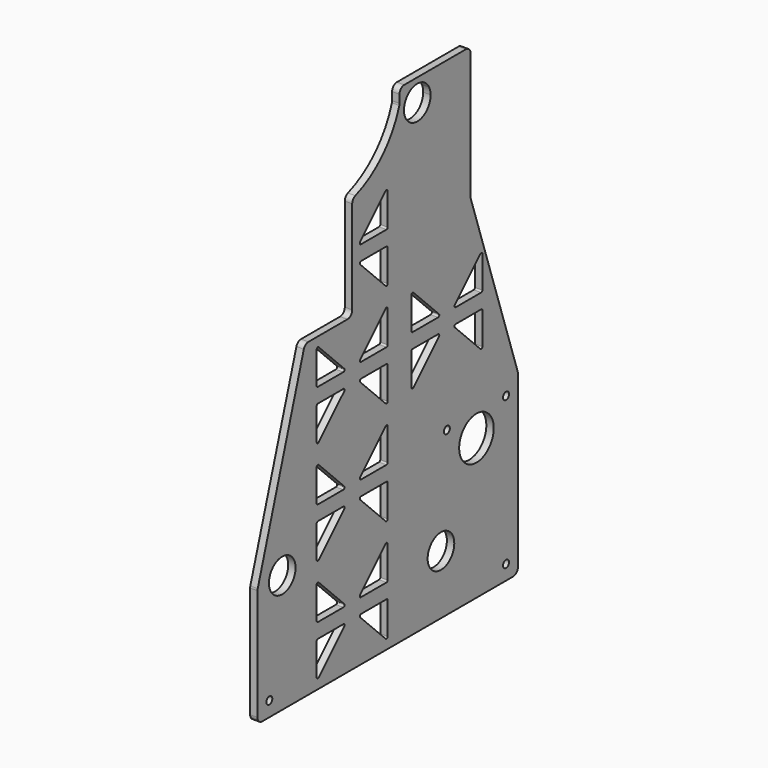
from build123d import *

# Parameters (mm, degrees)
F0_R     = 3.175
F0_R_2   = 14.2875
F0_R_3   = 18.542
F1_DEPTH = 6.35
F2_R     = 5.08
F3_R     = 5.08
F4_R     = 5.08


# Not quite as in the source:
# - two fillets or chamfers of one size are made in one step


with BuildPart() as f1:
    # F0 (on Right) → F1 (new body)
    with BuildSketch(Plane.YZ):
        with BuildLine():
            Line((0, 266.7), (0, 0))
            Line((0, 0), (101.6, 0))
            Line((101.6, 0), (101.6, 152.4))
            Line((101.6, 152.4), (101.6, 190.5))
            Line((101.6, 190.5), (101.6, 304.8))
            Line((101.6, 304.8), (101.6, 406.4))
            ThreePointArc((101.6, 406.4), (82.5624879144, 374.6375120856), (50.8, 355.6))
            Line((50.8, 355.6), (50.8, 266.7))
            Line((50.8, 266.7), (0, 266.7))
        make_face()
        with BuildLine():
            ThreePointArc((14.8680256121, 8.5180256121), (13.4839920409, 8.2427242179), (12.7, 9.4160512242))
            Line((12.7, 9.4160512242), (12.7, 36.83))
            ThreePointArc((12.7, 36.83), (13.0719743879, 37.7280256121), (13.97, 38.1))
            Line((13.97, 38.1), (41.3839487758, 38.1))
            ThreePointArc((41.3839487758, 38.1), (42.5572757821, 37.3160079591), (42.2819743879, 35.9319743879))
            Line((42.2819743879, 35.9319743879), (14.8680256121, 8.5180256121))
        make_face(mode=Mode.SUBTRACT)
        with BuildLine():
            Line((88.9, 36.83), (88.9, 9.4160512242))
            ThreePointArc((88.9, 9.4160512242), (88.1160079591, 8.2427242179), (86.7319743879, 8.5180256121))
            Line((86.7319743879, 8.5180256121), (59.3180256121, 35.9319743879))
            ThreePointArc((59.3180256121, 35.9319743879), (59.0427242179, 37.3160079591), (60.2160512242, 38.1))
            Line((60.2160512242, 38.1), (87.63, 38.1))
            ThreePointArc((87.63, 38.1), (88.5280256121, 37.7280256121), (88.9, 36.83))
        make_face(mode=Mode.SUBTRACT)
        with BuildLine():
            Line((41.3839487758, 50.8), (13.97, 50.8))
            ThreePointArc((13.97, 50.8), (13.0719743879, 51.1719743879), (12.7, 52.07))
            Line((12.7, 52.07), (12.7, 79.4839487758))
            ThreePointArc((12.7, 79.4839487758), (13.4839920409, 80.6572757821), (14.8680256121, 80.3819743879))
            Line((14.8680256121, 80.3819743879), (42.2819743879, 52.9680256121))
            ThreePointArc((42.2819743879, 52.9680256121), (42.5572757821, 51.5839920409), (41.3839487758, 50.8))
        make_face(mode=Mode.SUBTRACT)
        with BuildLine():
            ThreePointArc((60.2160512242, 50.8), (59.0427242179, 51.5839920409), (59.3180256121, 52.9680256121))
            Line((59.3180256121, 52.9680256121), (86.7319743879, 80.3819743879))
            ThreePointArc((86.7319743879, 80.3819743879), (88.1160079591, 80.6572757821), (88.9, 79.4839487758))
            Line((88.9, 79.4839487758), (88.9, 52.07))
            ThreePointArc((88.9, 52.07), (88.5280256121, 51.1719743879), (87.63, 50.8))
            Line((87.63, 50.8), (60.2160512242, 50.8))
        make_face(mode=Mode.SUBTRACT)
        with BuildLine():
            Line((12.7, 98.3160512242), (12.7, 125.73))
            ThreePointArc((12.7, 125.73), (13.0719743879, 126.6280256121), (13.97, 127))
            Line((13.97, 127), (41.3839487758, 127))
            ThreePointArc((41.3839487758, 127), (42.5572757821, 126.2160079591), (42.2819743879, 124.8319743879))
            Line((42.2819743879, 124.8319743879), (14.8680256121, 97.4180256121))
            ThreePointArc((14.8680256121, 97.4180256121), (13.4839920409, 97.1427242179), (12.7, 98.3160512242))
        make_face(mode=Mode.SUBTRACT)
        with BuildLine():
            Line((41.3839487758, 139.7), (13.97, 139.7))
            ThreePointArc((13.97, 139.7), (13.0719743879, 140.0719743879), (12.7, 140.97))
            Line((12.7, 140.97), (12.7, 168.3839487758))
            ThreePointArc((12.7, 168.3839487758), (13.4839920409, 169.5572757821), (14.8680256121, 169.2819743879))
            Line((14.8680256121, 169.2819743879), (42.2819743879, 141.8680256121))
            ThreePointArc((42.2819743879, 141.8680256121), (42.5572757821, 140.4839920409), (41.3839487758, 139.7))
        make_face(mode=Mode.SUBTRACT)
        with BuildLine():
            Line((88.9, 125.73), (88.9, 98.3160512242))
            ThreePointArc((88.9, 98.3160512242), (88.1160079591, 97.1427242179), (86.7319743879, 97.4180256121))
            Line((86.7319743879, 97.4180256121), (59.3180256121, 124.8319743879))
            ThreePointArc((59.3180256121, 124.8319743879), (59.0427242179, 126.2160079591), (60.2160512242, 127))
            Line((60.2160512242, 127), (87.63, 127))
            ThreePointArc((87.63, 127), (88.5280256121, 126.6280256121), (88.9, 125.73))
        make_face(mode=Mode.SUBTRACT)
        with BuildLine():
            ThreePointArc((60.2160512242, 139.7), (59.0427242179, 140.4839920409), (59.3180256121, 141.8680256121))
            Line((59.3180256121, 141.8680256121), (86.7319743879, 169.2819743879))
            ThreePointArc((86.7319743879, 169.2819743879), (88.1160079591, 169.5572757821), (88.9, 168.3839487758))
            Line((88.9, 168.3839487758), (88.9, 140.97))
            ThreePointArc((88.9, 140.97), (88.5280256121, 140.0719743879), (87.63, 139.7))
            Line((87.63, 139.7), (60.2160512242, 139.7))
        make_face(mode=Mode.SUBTRACT)
        with BuildLine():
            ThreePointArc((14.8680256121, 186.3180256121), (13.4839920409, 186.0427242179), (12.7, 187.2160512242))
            Line((12.7, 187.2160512242), (12.7, 214.63))
            ThreePointArc((12.7, 214.63), (13.0719743879, 215.5280256121), (13.97, 215.9))
            Line((13.97, 215.9), (41.3839487758, 215.9))
            ThreePointArc((41.3839487758, 215.9), (42.5572757821, 215.1160079591), (42.2819743879, 213.7319743879))
            Line((42.2819743879, 213.7319743879), (14.8680256121, 186.3180256121))
        make_face(mode=Mode.SUBTRACT)
        with BuildLine():
            Line((88.9, 214.63), (88.9, 187.2160512242))
            ThreePointArc((88.9, 187.2160512242), (88.1160079591, 186.0427242179), (86.7319743879, 186.3180256121))
            Line((86.7319743879, 186.3180256121), (59.3180256121, 213.7319743879))
            ThreePointArc((59.3180256121, 213.7319743879), (59.0427242179, 215.1160079591), (60.2160512242, 215.9))
            Line((60.2160512242, 215.9), (87.63, 215.9))
            ThreePointArc((87.63, 215.9), (88.5280256121, 215.5280256121), (88.9, 214.63))
        make_face(mode=Mode.SUBTRACT)
        with BuildLine():
            Line((41.3839487758, 228.6), (13.97, 228.6))
            ThreePointArc((13.97, 228.6), (13.0719743879, 228.9719743879), (12.7, 229.87))
            Line((12.7, 229.87), (12.7, 257.2839487758))
            ThreePointArc((12.7, 257.2839487758), (13.4839920409, 258.4572757821), (14.8680256121, 258.1819743879))
            Line((14.8680256121, 258.1819743879), (42.2819743879, 230.7680256121))
            ThreePointArc((42.2819743879, 230.7680256121), (42.5572757821, 229.3839920409), (41.3839487758, 228.6))
        make_face(mode=Mode.SUBTRACT)
        with BuildLine():
            ThreePointArc((60.2160512242, 228.6), (59.0427242179, 229.3839920409), (59.3180256121, 230.7680256121))
            Line((59.3180256121, 230.7680256121), (86.7319743879, 258.1819743879))
            ThreePointArc((86.7319743879, 258.1819743879), (88.1160079591, 258.4572757821), (88.9, 257.2839487758))
            Line((88.9, 257.2839487758), (88.9, 229.87))
            ThreePointArc((88.9, 229.87), (88.5280256121, 228.9719743879), (87.63, 228.6))
            Line((87.63, 228.6), (60.2160512242, 228.6))
        make_face(mode=Mode.SUBTRACT)
        with BuildLine():
            Line((88.9, 303.53), (88.9, 276.1160512242))
            ThreePointArc((88.9, 276.1160512242), (88.1160079591, 274.9427242179), (86.7319743879, 275.2180256121))
            Line((86.7319743879, 275.2180256121), (59.3180256121, 302.6319743879))
            ThreePointArc((59.3180256121, 302.6319743879), (59.0427242179, 304.0160079591), (60.2160512242, 304.8))
            Line((60.2160512242, 304.8), (87.63, 304.8))
            ThreePointArc((87.63, 304.8), (88.5280256121, 304.4280256121), (88.9, 303.53))
        make_face(mode=Mode.SUBTRACT)
        with BuildLine():
            Line((87.63, 317.5), (60.2160512242, 317.5))
            ThreePointArc((60.2160512242, 317.5), (59.0427242179, 318.2839920409), (59.3180256121, 319.6680256121))
            Line((59.3180256121, 319.6680256121), (86.7319743879, 347.0819743879))
            ThreePointArc((86.7319743879, 347.0819743879), (88.1160079591, 347.3572757821), (88.9, 346.1839487758))
            Line((88.9, 346.1839487758), (88.9, 318.77))
            ThreePointArc((88.9, 318.77), (88.5280256121, 317.8719743879), (87.63, 317.5))
        make_face(mode=Mode.SUBTRACT)
        Polygon((-50.8, 0), (0, 0), (0, 266.7), (-50.8, 101.6), align=None)
        with Locations((-38.1, 12.7)):
            Circle(F0_R, mode=Mode.SUBTRACT)
        with Locations((-24.24176, 101.6)):
            Circle(F0_R_2, mode=Mode.SUBTRACT)
        Polygon((101.6, 152.4), (101.6, 0), (228.6, 0), (228.6, 152.4), (139.7, 152.4), align=None)
        with Locations((146.05, 50.8)):
            Circle(F0_R_2, mode=Mode.SUBTRACT)
        with Locations((215.9, 12.7)):
            Circle(F0_R, mode=Mode.SUBTRACT)
        with Locations((152.4, 139.7)):
            Circle(F0_R, mode=Mode.SUBTRACT)
        with Locations((184.15, 120.65)):
            Circle(F0_R_3, mode=Mode.SUBTRACT)
        with Locations((215.9, 139.7)):
            Circle(F0_R, mode=Mode.SUBTRACT)
        with BuildLine():
            Line((101.6, 190.5), (101.6, 152.4))
            Line((101.6, 152.4), (139.7, 152.4))
            ThreePointArc((139.7, 152.4), (112.7592316368, 163.5592316368), (101.6, 190.5))
        make_face()
        with BuildLine():
            Line((101.6, 304.8), (101.6, 190.5))
            ThreePointArc((101.6, 190.5), (112.7592316368, 163.5592316368), (139.7, 152.4))
            Line((139.7, 152.4), (228.6, 152.4))
            Line((228.6, 152.4), (177.8, 304.8))
            Line((177.8, 304.8), (101.6, 304.8))
        make_face()
        with BuildLine():
            Line((114.3, 187.2160512242), (114.3, 190.5))
            Line((114.3, 190.5), (114.3, 214.63))
            ThreePointArc((114.3, 214.63), (114.6719743879, 215.5280256121), (115.57, 215.9))
            Line((115.57, 215.9), (142.9839487758, 215.9))
            ThreePointArc((142.9839487758, 215.9), (144.1572757821, 215.1160079591), (143.8819743879, 213.7319743879))
            Line((143.8819743879, 213.7319743879), (120.65, 190.5))
            Line((120.65, 190.5), (116.4680256121, 186.3180256121))
            ThreePointArc((116.4680256121, 186.3180256121), (115.0839920409, 186.0427242179), (114.3, 187.2160512242))
        make_face(mode=Mode.SUBTRACT)
        with BuildLine():
            ThreePointArc((189.23, 215.9), (190.1280256121, 215.5280256121), (190.5, 214.63))
            Line((190.5, 214.63), (190.5, 187.2160512242))
            ThreePointArc((190.5, 187.2160512242), (189.7160079591, 186.0427242179), (188.3319743879, 186.3180256121))
            Line((188.3319743879, 186.3180256121), (160.9180256121, 213.7319743879))
            ThreePointArc((160.9180256121, 213.7319743879), (160.6427242179, 215.1160079591), (161.8160512242, 215.9))
            Line((161.8160512242, 215.9), (189.23, 215.9))
        make_face(mode=Mode.SUBTRACT)
        with BuildLine():
            ThreePointArc((115.57, 228.6), (114.6719743879, 228.9719743879), (114.3, 229.87))
            Line((114.3, 229.87), (114.3, 257.2839487758))
            ThreePointArc((114.3, 257.2839487758), (115.0839920409, 258.4572757821), (116.4680256121, 258.1819743879))
            Line((116.4680256121, 258.1819743879), (143.8819743879, 230.7680256121))
            ThreePointArc((143.8819743879, 230.7680256121), (144.1572757821, 229.3839920409), (142.9839487758, 228.6))
            Line((142.9839487758, 228.6), (115.57, 228.6))
        make_face(mode=Mode.SUBTRACT)
        with BuildLine():
            Line((190.5, 257.2839487758), (190.5, 229.87))
            ThreePointArc((190.5, 229.87), (190.1280256121, 228.9719743879), (189.23, 228.6))
            Line((189.23, 228.6), (161.8160512242, 228.6))
            ThreePointArc((161.8160512242, 228.6), (160.6427242179, 229.3839920409), (160.9180256121, 230.7680256121))
            Line((160.9180256121, 230.7680256121), (188.3319743879, 258.1819743879))
            ThreePointArc((188.3319743879, 258.1819743879), (189.7160079591, 258.4572757821), (190.5, 257.2839487758))
        make_face(mode=Mode.SUBTRACT)
        with BuildLine():
            Line((101.6, 406.4), (101.6, 304.8))
            Line((101.6, 304.8), (177.8, 304.8))
            Line((177.8, 304.8), (177.8, 406.4))
            Line((177.8, 406.4), (133.4488341754, 406.4))
            ThreePointArc((133.4488341754, 406.4), (134.5603558461, 403.3110821033), (134.9375, 400.05))
            ThreePointArc((134.9375, 400.05), (117.3889178967, 386.1396441539), (107.8511658246, 406.4))
            Line((107.8511658246, 406.4), (101.6, 406.4))
        make_face()
        with BuildLine():
            Line((101.6, 419.1), (101.6, 406.4))
            Line((101.6, 406.4), (107.8511658246, 406.4))
            ThreePointArc((107.8511658246, 406.4), (120.65, 414.3375), (133.4488341754, 406.4))
            Line((133.4488341754, 406.4), (177.8, 406.4))
            Line((177.8, 406.4), (177.8, 419.1))
            Line((177.8, 419.1), (101.6, 419.1))
        make_face()
    extrude(amount=F1_DEPTH)

    # F2
    f2_edges = [f1.edges().sort_by_distance(p)[0] for p in [
        (3.175, 101.6, 406.4),
        (3.175, 101.6, 419.1),
        (3.175, 177.8, 419.1),
    ]]
    fillet(f2_edges, radius=F2_R)

    # F3
    f3_edges = [f1.edges().sort_by_distance(p)[0] for p in [
        (3.175, 0, 266.7),
        (3.175, 50.8, 266.7),
    ]]
    fillet(f3_edges, radius=F3_R)

    # F4
    f4_edges = [f1.edges().sort_by_distance(p)[0] for p in [
        (3.175, 50.8, 355.6),
        (3.175, -50.8, 101.6),
        (3.175, -50.8, 0),
        (3.175, 228.6, 0),
        (3.175, 228.6, 152.4),
        (3.175, 177.8, 304.8),
    ]]
    fillet(f4_edges, radius=F4_R)


solid = f1.part
